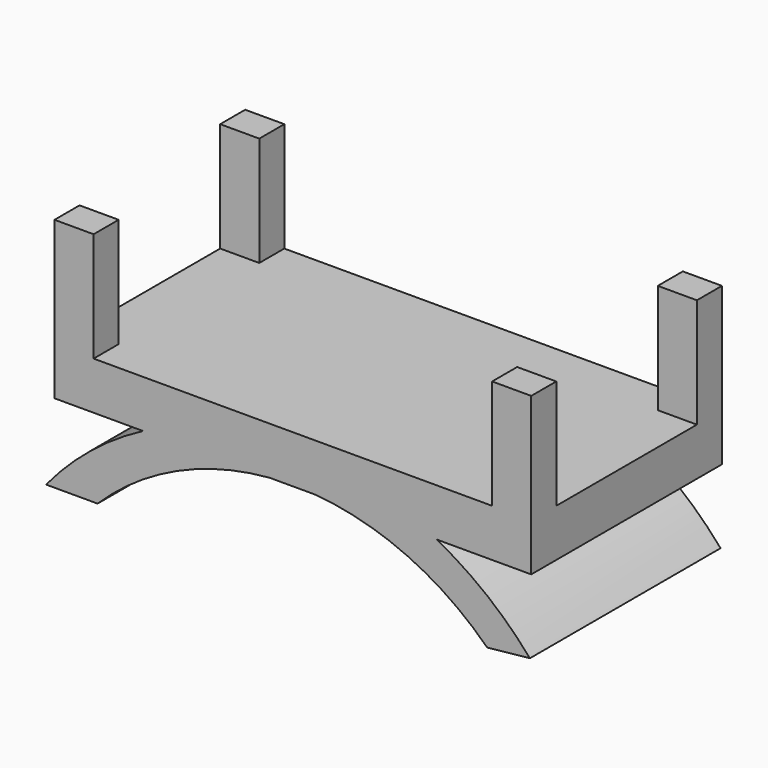
from build123d import *

# Parameters (mm, degrees)
F0_W     = 304.8
F0_H     = 30.48
F1_DEPTH = 152.4
F2_W     = 25
F2_H     = 20
F3_DEPTH = 70
F5_DEPTH = 152.4


# Not quite as in the source:
# - the program builds the solid bodies; features that only make, move or delete a surface that nothing else refers to are left out


with BuildPart() as f1:
    # F0 (on Front) → F1 (new body)
    with BuildSketch(Plane.XZ):
        Rectangle(F0_W, F0_H)
    extrude(amount=F1_DEPTH)

    # F2 (on face) → F3 (join)
    with BuildSketch(Plane.XY.offset(15.24)):
        with Locations((-139.9, -10)):
            Rectangle(F2_W, F2_H)
        with Locations((-139.9, -142.4)):
            Rectangle(F2_W, F2_H)
        with Locations((139.9, -10)):
            Rectangle(F2_W, F2_H)
        with Locations((139.9, -142.4)):
            Rectangle(F2_W, F2_H)
    extrude(amount=F3_DEPTH)

    # F4 (on Front) → F5 (join)
    with BuildSketch(Plane.XZ):
        with BuildLine():
            Line((124.2321878223, -65.5579566956), (151.5389296347, -62.7254612585))
            ThreePointArc((151.5389296347, -62.7254612585), (-3.7822030549, 7.8738857172), (-157.7844321728, -65.5579566956))
            Line((-157.7844321728, -65.5579566956), (-124.8654021339, -65.5579566956))
            ThreePointArc((-124.8654021339, -65.5579566956), (-0.3166071558, -14.6454567478), (124.2321878223, -65.5579566956))
        make_face()
    extrude(amount=F5_DEPTH)


solid = f1.part
